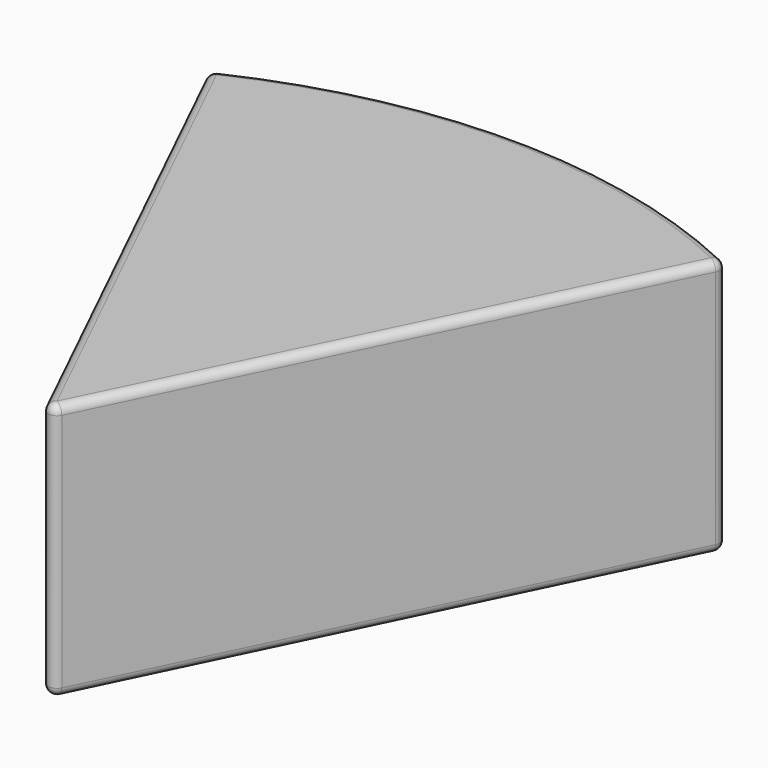
from build123d import *

# Parameters (mm, degrees)
F1_DEPTH = 19.05
F3_R     = 1.27


# Not quite as in the source:
# - a feature of the source that left no trace in its solid (it failed there, or was rolled back) is left out


with BuildPart() as f1:
    # F0 (on Top) → F1 (new body, symmetric)
    with BuildSketch(Plane.XY):
        with BuildLine():
            Line((-38.3560955603, 23.021564283), (0, -55.7964481413))
            Line((0, -55.7964481413), (38.3560955603, 23.021564283))
            ThreePointArc((38.3560955603, 23.021564283), (0, 31.8589518587), (-38.3560955603, 23.021564283))
        make_face()
    extrude(amount=F1_DEPTH, both=True)

    # F3
    f3_edges = [f1.edges().sort_by_distance(p)[0] for p in [
        (0, -55.796448, 0),
        (38.356096, 23.021564, 0),
        (-38.356096, 23.021564, 0),
        (-19.178048, -16.387442, -19.05),
        (-19.178048, -16.387442, 19.05),
        (0, 31.858952, -19.05),
        (0, 31.858952, 19.05),
        (19.178048, -16.387442, 19.05),
        (19.178048, -16.387442, -19.05),
    ]]
    fillet(f3_edges, radius=F3_R)


solid = f1.part
